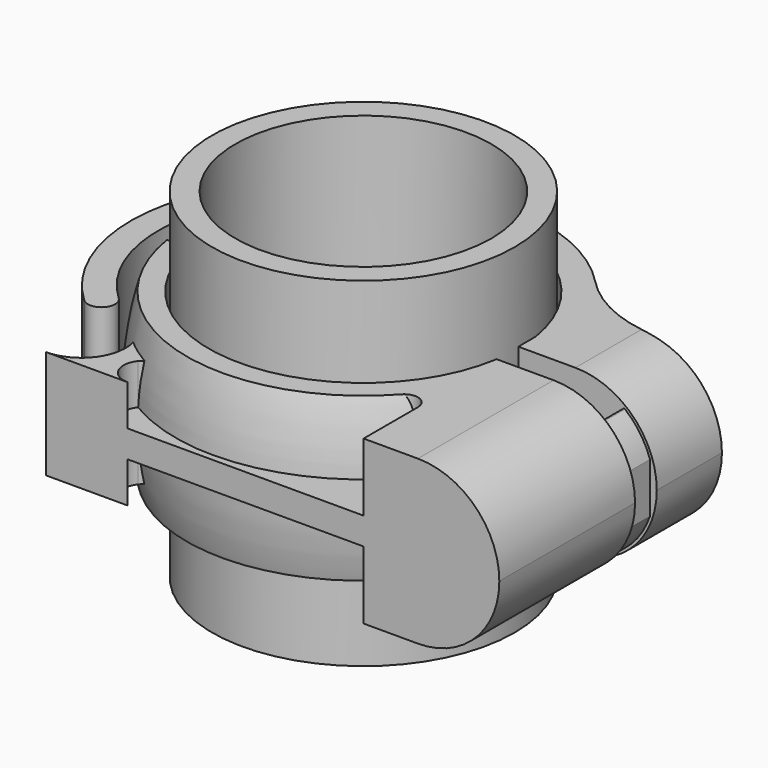
from build123d import *

# Parameters (mm, degrees)
F0_R      = 11.15
F0_R_2    = 9.4288540256
F1_DEPTH  = 12.5
F4_DEPTH  = 6
F6_DEPTH  = 1
F7_DEPTH  = 4
F8_R      = 5.99999
F9_START  = 2
F9_DEPTH  = 6
F11_DEPTH = 2
F12_R     = 0.1
F10_R     = 1.5
F13_DEPTH = 7.6
F15_DEPTH = 6
F16_R     = 10
F17_R     = 2
F18_DEPTH = 25


# Not quite as in the source:
# - a fillet or chamfer is up to 0.001 mm smaller than in the source, because OpenCascade refuses the exact size


with BuildPart() as f1:
    # F0 (on Top) → F1 (new body, symmetric)
    with BuildSketch(Plane.XY):
        Circle(F0_R)
        Circle(F0_R_2, mode=Mode.SUBTRACT)
    extrude(amount=F1_DEPTH, both=True)


with BuildPart() as f4:
    # F2 (on Top) → F4 (new body, symmetric)
    with BuildSketch(Plane.XY):
        with BuildLine():
            ThreePointArc((11.2569978236, -1.8), (0, -11.4), (-11.2569978236, -1.8))
            Line((-11.2569978236, -1.8), (-12.8369273427, -2.0526315789))
            ThreePointArc((-12.8369273427, -2.0526315789), (-11.6914767069, -5.6841333915), (-9.5429207129, -8.827947908))
            ThreePointArc((-9.5429207129, -8.827947908), (-8.0364228667, -10.2184102241), (-6.3300643569, -11.3547472555))
            ThreePointArc((-6.3300643569, -11.3547472555), (2.1664427623, -12.8182107081), (9.7100694076, -8.6437579848))
            ThreePointArc((9.7100694076, -8.6437579848), (10.3065484867, -8.3200447248), (10.9723211553, -8.4516666087))
            ThreePointArc((10.9723211553, -8.4516666087), (11.3274354525, -8.8163837293), (11.4569978236, -9.3086624451))
            Line((11.4569978236, -9.3086624451), (11.4569978236, -14.3))
            Line((11.4569978236, -14.3), (21.4569978236, -14.3))
            Line((21.4569978236, -14.3), (21.4569978236, -1.8))
            Line((21.4569978236, -1.8), (11.2569978236, -1.8))
        make_face()
    extrude(amount=F4_DEPTH, both=True)

    # F5: sweep along a path in F2
    with BuildLine(Plane.XY) as f5_path:
        ThreePointArc((-13.6762648997, -2.1868421053), (-3.4117201611, -13.4232136816), (10.9723211553, -8.4516666087))
    # F3 (on Right) → F5 (sweep)
    with BuildSketch(Plane.YZ):
        with BuildLine():
            Line((-11.4, -6), (-11.4, 6))
            Line((-11.4, 6), (-13, 6))
            ThreePointArc((-13, 6), (-13.85, 0), (-13, -6))
            Line((-13, -6), (-11.4, -6))
        make_face()
    sweep(path=f5_path.line)

    # F2 (on Top) → F6 (join, symmetric)
    with BuildSketch(Plane.XY):
        with BuildLine():
            Line((-5.9285117394, -14.3), (11.4569978236, -14.3))
            Line((11.4569978236, -14.3), (11.4569978236, -9.3086624451))
            ThreePointArc((11.4569978236, -9.3086624451), (11.3274354525, -8.8163837293), (10.9723211553, -8.4516666087))
            ThreePointArc((10.9723211553, -8.4516666087), (2.5810942069, -13.6073675887), (-7.1152481611, -11.8825815211))
            ThreePointArc((-7.1152481611, -11.8825815211), (-7.2750123369, -13.4610114529), (-5.9285117394, -14.3))
        make_face()
        with BuildLine():
            ThreePointArc((9.7100694076, -8.6437579848), (2.1664427623, -12.8182107081), (-6.3300643569, -11.3547472555))
            ThreePointArc((-6.3300643569, -11.3547472555), (-6.7653616489, -11.5551376667), (-7.1152481611, -11.8825815211))
            ThreePointArc((-7.1152481611, -11.8825815211), (2.5810942069, -13.6073675887), (10.9723211553, -8.4516666087))
            ThreePointArc((10.9723211553, -8.4516666087), (10.3065484867, -8.3200447248), (9.7100694076, -8.6437579848))
        make_face()
        with BuildLine():
            ThreePointArc((-6.3300643569, -11.3547472555), (-8.0364228667, -10.2184102241), (-9.5429207129, -8.827947908))
            ThreePointArc((-9.5429207129, -8.827947908), (-8.9491796093, -9.7355161295), (-8.6861285989, -10.7876628592))
            ThreePointArc((-8.6861285989, -10.7876628592), (-7.91963311, -11.3623022052), (-7.1152481611, -11.8825815211))
            ThreePointArc((-7.1152481611, -11.8825815211), (-6.7653616489, -11.5551376667), (-6.3300643569, -11.3547472555))
        make_face()
        with BuildLine():
            ThreePointArc((-7.1152481611, -11.8825815211), (-7.91963311, -11.3623022052), (-8.6861285989, -10.7876628592))
            ThreePointArc((-8.6861285989, -10.7876628592), (-9.5428942517, -13.2540789242), (-11.9352371812, -14.3))
            Line((-11.9352371812, -14.3), (-5.9285117394, -14.3))
            ThreePointArc((-5.9285117394, -14.3), (-7.2750123369, -13.4610114529), (-7.1152481611, -11.8825815211))
        make_face()
    extrude(amount=F6_DEPTH, both=True)

    # F2 (on Top) → F7 (join, symmetric)
    with BuildSketch(Plane.XY):
        with BuildLine():
            ThreePointArc((-6.3300643569, -11.3547472555), (-8.0364228667, -10.2184102241), (-9.5429207129, -8.827947908))
            ThreePointArc((-9.5429207129, -8.827947908), (-8.9491796093, -9.7355161295), (-8.6861285989, -10.7876628592))
            ThreePointArc((-8.6861285989, -10.7876628592), (-7.91963311, -11.3623022052), (-7.1152481611, -11.8825815211))
            ThreePointArc((-7.1152481611, -11.8825815211), (-6.7653616489, -11.5551376667), (-6.3300643569, -11.3547472555))
        make_face()
        with BuildLine():
            ThreePointArc((-7.1152481611, -11.8825815211), (-7.91963311, -11.3623022052), (-8.6861285989, -10.7876628592))
            ThreePointArc((-8.6861285989, -10.7876628592), (-9.5428942517, -13.2540789242), (-11.9352371812, -14.3))
            Line((-11.9352371812, -14.3), (-5.9285117394, -14.3))
            ThreePointArc((-5.9285117394, -14.3), (-7.2750123369, -13.4610114529), (-7.1152481611, -11.8825815211))
        make_face()
    extrude(amount=F7_DEPTH, both=True)

    # F8 (radius 6 in the source; OpenCascade refuses exactly that, so slightly less here)
    f8_edges = [f4.edges().sort_by_distance(p)[0] for p in [
        (21.456998, -8.05, 6),
        (21.456998, -8.05, -6),
    ]]
    fillet(f8_edges, radius=F8_R)

    # F10 (on face) → F11 (join)
    with BuildSketch(Plane(origin=(0, -1.8, 0), x_dir=(-1, 0, 0), z_dir=(0, 1, 0))):
        with BuildLine():
            Line((-18.9569978236, -4.6249324319), (-18.9569978236, 4.6249324319))
            ThreePointArc((-18.9569978236, 4.6249324319), (-20.1673373183, 3.3841840737), (-20.9569978236, 1.841195264))
            Line((-20.9569978236, 1.841195264), (-20.9569978236, -1.841195264))
            ThreePointArc((-20.9569978236, -1.841195264), (-20.1673373183, -3.3841840737), (-18.9569978236, -4.6249324319))
        make_face()
    extrude(amount=F11_DEPTH)

    # F12
    f12_edges = [f4.edges().sort_by_distance(p)[0] for p in [
        (18.956998, -0.8, 4.624932),
        (18.956998, -0.8, -4.624932),
    ]]
    fillet(f12_edges, radius=F12_R)

    # F10 (on face) → F13 (cut)
    with BuildSketch(Plane(origin=(0, -1.8, 0), x_dir=(-1, 0, 0), z_dir=(0, 1, 0))):
        with Locations((-15.4569978236, 0)):
            Circle(F10_R)
    extrude(amount=-F13_DEPTH, mode=Mode.SUBTRACT)


with BuildPart() as f9:
    # F4_face (on face) → F9 (new body)
    with BuildSketch(Plane(origin=(15.8138062617, -1.8, 0), x_dir=(-1, 0, 0), z_dir=(0, 1, 0)).offset(F9_START)):
        with BuildLine():
            Line((-5.6431915618, 1e-05), (-5.6431915618, -1e-05))
            ThreePointArc((-5.6431915618, -1e-05), (-3.8858351779, -4.2426436161), (0.3567984382, -6))
            Line((0.3567984382, -6), (4.5568084382, -6))
            Line((4.5568084382, -6), (4.5568084382, 6))
            Line((4.5568084382, 6), (0.3567984382, 6))
            ThreePointArc((0.3567984382, 6), (-3.8858351779, 4.2426436161), (-5.6431915618, 1e-05))
        make_face()
    extrude(amount=F9_DEPTH)

    # F14 (on Top) → F15 (join, symmetric)
    with BuildSketch(Plane.XY):
        with BuildLine():
            ThreePointArc((0, 11.4), (7.9899937422, 8.1314205401), (11.398245479, 0.2))
            Line((11.398245479, 0.2), (13.3985073796, 0.2))
            ThreePointArc((13.3985073796, 0.2), (9.4042543564, 9.545679651), (0, 13.4))
            ThreePointArc((0, 13.4), (-8.8214702408, 10.7963483499), (-14.8153922738, 3.8199425569))
            ThreePointArc((-14.8153922738, 3.8199425569), (-15.6943952458, -4.017992702), (-11.8403594103, -10.8992922251))
            ThreePointArc((-11.8403594103, -10.8992922251), (-10.4270753871, -10.8480255729), (-10.4783420392, -9.4347415497))
            ThreePointArc((-10.4783420392, -9.4347415497), (-13.3483970384, -5.0332308443), (-13.8214796077, 0.2))
            ThreePointArc((-13.8214796077, 0.2), (-13.5007989075, 1.6276240681), (-12.9914994214, 2.9993239714))
            ThreePointArc((-12.9914994214, 2.9993239714), (-7.7354769561, 9.1168786164), (0, 11.4))
        make_face()
        with BuildLine():
            ThreePointArc((-11.398245479, 0.2), (-7.9899937422, 8.1314205401), (0, 11.4))
            ThreePointArc((0, 11.4), (-7.7354769561, 9.1168786164), (-12.9914994214, 2.9993239714))
            ThreePointArc((-12.9914994214, 2.9993239714), (-13.5007989075, 1.6276240681), (-13.8214796077, 0.2))
            Line((-13.8214796077, 0.2), (-11.398245479, 0.2))
        make_face()
    extrude(amount=F15_DEPTH, both=True)

    # F16
    f16_edges = [f9.edges().sort_by_distance(p)[0] for p in [
        (11.879394, 6.2, 0),
    ]]
    fillet(f16_edges, radius=F16_R)

    # F17 (on face) → F18 (cut)
    with BuildSketch(Plane.XZ.offset(-0.2)):
        with Locations((15.4569978236, 0)):
            Circle(F17_R)
    extrude(amount=-F18_DEPTH, mode=Mode.SUBTRACT)


solid = Compound([f1.part, f4.part, f9.part])
